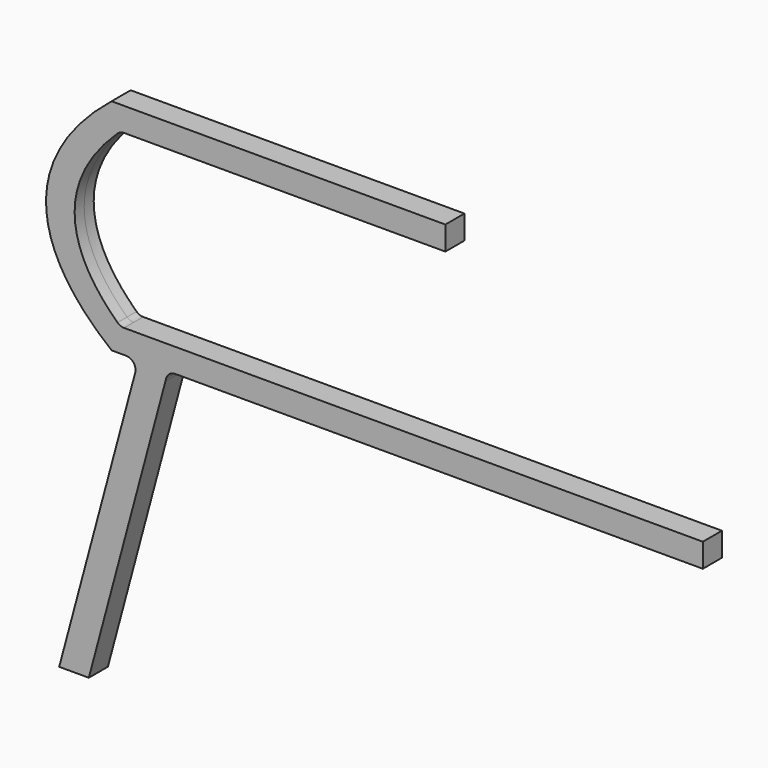
from build123d import *

# Parameters (mm, degrees)
F1_DEPTH = 12.5
F2_R     = 10


with BuildPart() as f1:
    # F0 (on Front) → F1 (new body, symmetric)
    with BuildSketch(Plane.XZ):
        with BuildLine():
            Line((350, 230), (40.9729498071, 230))
            add(Edge.make_bspline(
                [(40.9729498071, 230), (23.1266754436, 217.7466324391), (9.1600259417, 205)],
                knots=[5.8517425134, 5.8517425134, 5.8517425134, 5.949769397, 5.949769397, 5.949769397], degree=2, weights=[1, 0.9987990817, 1]))
            Line((9.1600259417, 205), (350, 205))
            Line((350, 205), (350, 230))
        make_face()
        with BuildLine():
            add(Edge.make_bspline(
                [(-68.7509398502, 115), (-68.7509398502, 55.2165740433), (0, 0)],
                knots=[0, 0, 0, 0.393402632, 0.393402632, 0.393402632], degree=2, weights=[1, 0.9807165918, 1]))
            Line((0, 0), (28.125, 0))
            Line((28.125, 0), (40.9729498071, 0))
            add(Edge.make_bspline(
                [(9.1600259417, 25), (23.1266754436, 12.2533675609), (40.9729498071, 0)],
                knots=[0.3334159102, 0.3334159102, 0.3334159102, 0.4314427937, 0.4314427937, 0.4314427937], degree=2, weights=[1, 0.9987990817, 1]))
            add(Edge.make_bspline(
                [(-38.7509398502, 115), (-38.7509398502, 68.7258392336), (9.1600259417, 25)],
                knots=[0, 0, 0, 0.3334159102, 0.3334159102, 0.3334159102], degree=2, weights=[1, 0.9861363811, 1]))
            add(Edge.make_bspline(
                [(9.1600259417, 205), (-38.7509398502, 161.2741607664), (-38.7509398502, 115)],
                knots=[5.949769397, 5.949769397, 5.949769397, 6.2831853072, 6.2831853072, 6.2831853072], degree=2, weights=[1, 0.9861363811, 1]))
            add(Edge.make_bspline(
                [(40.9729498071, 230), (23.1266754436, 217.7466324391), (9.1600259417, 205)],
                knots=[5.8517425134, 5.8517425134, 5.8517425134, 5.949769397, 5.949769397, 5.949769397], degree=2, weights=[1, 0.9987990817, 1]))
            Line((40.9729498071, 230), (0, 230))
            add(Edge.make_bspline(
                [(0, 230), (-68.7509398502, 174.7834259567), (-68.7509398502, 115)],
                knots=[5.8897826752, 5.8897826752, 5.8897826752, 6.2831853072, 6.2831853072, 6.2831853072], degree=2, weights=[1, 0.9807165918, 1]))
        make_face()
        with BuildLine():
            add(Edge.make_bspline(
                [(9.1600259417, 25), (23.1266754436, 12.2533675609), (40.9729498071, 0)],
                knots=[0.3334159102, 0.3334159102, 0.3334159102, 0.4314427937, 0.4314427937, 0.4314427937], degree=2, weights=[1, 0.9987990817, 1]))
            Line((40.9729498071, 0), (59.1832854123, 0))
            Line((59.1832854123, 0), (620, 0))
            Line((620, 0), (620, 25))
            Line((620, 25), (9.1600259417, 25))
        make_face()
        with BuildLine():
            Line((40.9729498071, 0), (28.125, 0))
            Line((28.125, 0), (23.4899694027, -17.2981696839))
            add(Edge.make_bspline(
                [(23.4899694027, -17.2981696839), (35.9947939251, -25.7814361907), (50.0769032841, -33.9854807757)],
                knots=[0.4567057683, 0.4567057683, 0.4567057683, 0.5196982713, 0.5196982713, 0.5196982713], degree=2, weights=[1, 0.9995040341, 1]))
            Line((50.0769032841, -33.9854807757), (56.4775823084, -10.0978214541))
            add(Edge.make_bspline(
                [(40.9729498071, 0), (48.3992260092, -5.0989293373), (56.4775823084, -10.0978214541)],
                knots=[0.4314427937, 0.4314427937, 0.4314427937, 0.4722612324, 0.4722612324, 0.4722612324], degree=2, weights=[1, 0.9997917391, 1]))
        make_face()
        with BuildLine():
            add(Edge.make_bspline(
                [(23.4899694027, -17.2981696839), (35.9947939251, -25.7814361907), (50.0769032841, -33.9854807757)],
                knots=[0.4567057683, 0.4567057683, 0.4567057683, 0.5196982713, 0.5196982713, 0.5196982713], degree=2, weights=[1, 0.9995040341, 1]))
            Line((23.4899694027, -17.2981696839), (-54.9392496536, -310))
            Line((-54.9392496536, -310), (-23.8809642413, -310))
            Line((-23.8809642413, -310), (50.0769032841, -33.9854807757))
        make_face()
        with BuildLine():
            Line((59.1832854123, 0), (40.9729498071, 0))
            add(Edge.make_bspline(
                [(40.9729498071, 0), (48.3992260092, -5.0989293373), (56.4775823084, -10.0978214541)],
                knots=[0.4314427937, 0.4314427937, 0.4314427937, 0.4722612324, 0.4722612324, 0.4722612324], degree=2, weights=[1, 0.9997917391, 1]))
            Line((56.4775823084, -10.0978214541), (59.1832854123, 0))
        make_face()
    extrude(amount=F1_DEPTH, both=True)

    # F2
    f2_edges = [f1.edges().sort_by_distance(p)[0] for p in [
        (9.160026, 6.25, 25),
        (9.160026, -6.25, 25),
        (9.160026, 6.25, 205),
        (9.160026, -6.25, 205),
        (59.183285, 0, 0),
        (28.125, 0, 0),
    ]]
    fillet(f2_edges, radius=F2_R)


solid = f1.part
